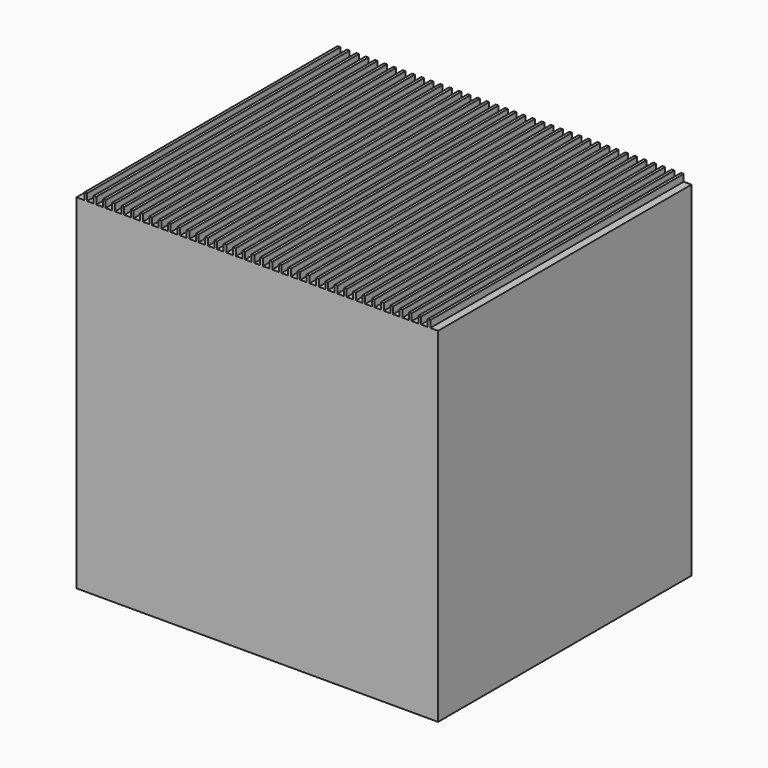
from build123d import *

# Parameters (mm, degrees)
F2_W         = 10.5
F2_H         = 9.2
F3_DEPTH     = 10
F4_W         = 0.08
F4_H         = 9.2
F5_DEPTH     = 0.2
F6_TEXT_SIZE = 7.3553824543
F7_DEPTH     = 2


# Not quite as in the source:
# - Text() gives the source's letters only with a copy of the font that has no kerning and outlines rounded to 1/6400 em; it was checked with that copy


with BuildPart() as f3:
    # F2 (on Top) → F3 (new body)
    with BuildSketch(Plane.XY):
        Rectangle(F2_W, F2_H)
    extrude(amount=F3_DEPTH)

    # F4 (on face) → F5 (join)
    with BuildSketch(Plane.XY.offset(10)):
        with Locations((0.125, 0)):
            Rectangle(F4_W, F4_H)
        with Locations((0.395, 0)):
            Rectangle(F4_W, F4_H)
        with Locations((0.665, 0)):
            Rectangle(F4_W, F4_H)
        with Locations((0.935, 0)):
            Rectangle(F4_W, F4_H)
        with Locations((1.205, 0)):
            Rectangle(F4_W, F4_H)
        with Locations((1.475, 0)):
            Rectangle(F4_W, F4_H)
        with Locations((1.745, 0)):
            Rectangle(F4_W, F4_H)
        with Locations((2.015, 0)):
            Rectangle(F4_W, F4_H)
        with Locations((2.285, 0)):
            Rectangle(F4_W, F4_H)
        with Locations((2.555, 0)):
            Rectangle(F4_W, F4_H)
        with Locations((2.825, 0)):
            Rectangle(F4_W, F4_H)
        with Locations((3.095, 0)):
            Rectangle(F4_W, F4_H)
        with Locations((3.365, 0)):
            Rectangle(F4_W, F4_H)
        with Locations((3.635, 0)):
            Rectangle(F4_W, F4_H)
        with Locations((3.905, 0)):
            Rectangle(F4_W, F4_H)
        with Locations((4.175, 0)):
            Rectangle(F4_W, F4_H)
        with Locations((4.445, 0)):
            Rectangle(F4_W, F4_H)
        with Locations((4.715, 0)):
            Rectangle(F4_W, F4_H)
        with Locations((4.985, 0)):
            Rectangle(F4_W, F4_H)
        with Locations((-0.395, 0)):
            Rectangle(F4_W, F4_H)
        with Locations((-0.125, 0)):
            Rectangle(F4_W, F4_H)
        with Locations((-4.715, 0)):
            Rectangle(F4_W, F4_H)
        with Locations((-2.555, 0)):
            Rectangle(F4_W, F4_H)
        with Locations((-3.635, 0)):
            Rectangle(F4_W, F4_H)
        with Locations((-1.745, 0)):
            Rectangle(F4_W, F4_H)
        with Locations((-2.015, 0)):
            Rectangle(F4_W, F4_H)
        with Locations((-1.475, 0)):
            Rectangle(F4_W, F4_H)
        with Locations((-4.985, 0)):
            Rectangle(F4_W, F4_H)
        with Locations((-3.365, 0)):
            Rectangle(F4_W, F4_H)
        with Locations((-0.935, 0)):
            Rectangle(F4_W, F4_H)
        with Locations((-4.445, 0)):
            Rectangle(F4_W, F4_H)
        with Locations((-2.825, 0)):
            Rectangle(F4_W, F4_H)
        with Locations((-3.905, 0)):
            Rectangle(F4_W, F4_H)
        with Locations((-3.095, 0)):
            Rectangle(F4_W, F4_H)
        with Locations((-4.175, 0)):
            Rectangle(F4_W, F4_H)
        with Locations((-1.205, 0)):
            Rectangle(F4_W, F4_H)
        with Locations((-2.285, 0)):
            Rectangle(F4_W, F4_H)
        with Locations((-0.665, 0)):
            Rectangle(F4_W, F4_H)
    extrude(amount=F5_DEPTH)

    # F6 (on face) → F7 (cut)
    with BuildSketch(Plane(origin=(0, 0, 0), x_dir=(1, 0, 0), z_dir=(0, 0, -1))):
        with Locations((-4.4551175714, -2.50486086)):
            Text('1b', F6_TEXT_SIZE, font='Open Sans', font_style=FontStyle.BOLD, text_align=(TextAlign.LEFT, TextAlign.BOTTOM))
    extrude(amount=-F7_DEPTH, mode=Mode.SUBTRACT)


solid = f3.part
